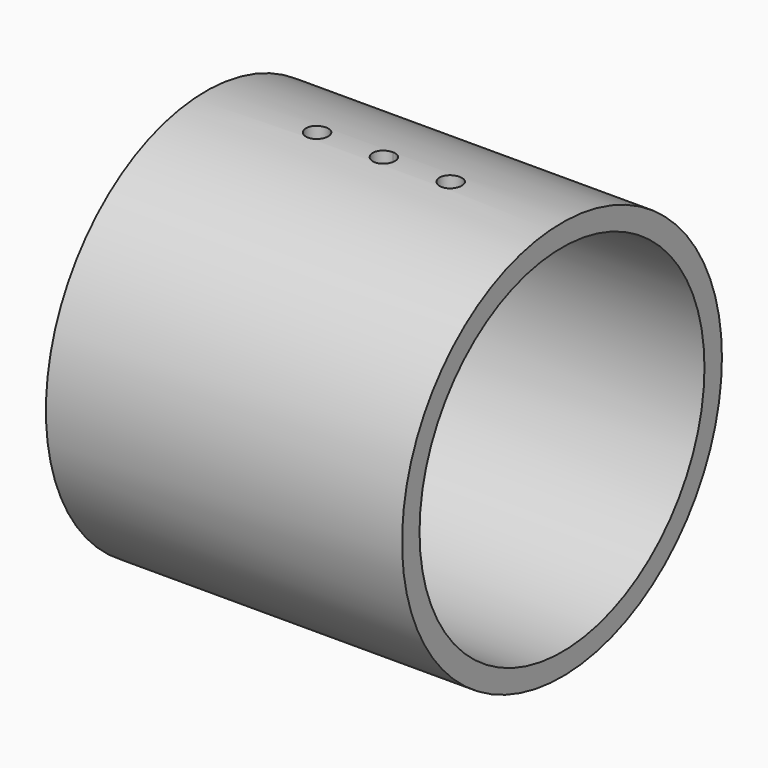
from build123d import *

# Parameters (mm, degrees)
F0_R     = 57.023
F0_R_2   = 50.8
F1_DEPTH = 101.6
F3_DEPTH = 127


# Not quite as in the source:
# - a pattern or mirror of a feature is missing from the dataset's text; its kind, count and spacing are read off the source's solid


with BuildPart() as f1:
    # F0 (on Right) → F1 (new body)
    with BuildSketch(Plane.YZ):
        Circle(F0_R)
        Circle(F0_R_2, mode=Mode.SUBTRACT)
    extrude(amount=F1_DEPTH)

    # F2 (on Top) → F3 (cut)
    with BuildSketch(Plane.XY):
        with BuildLine():
            ThreePointArc((53.975, 0), (50.8, 3.175), (47.625, 0))
            Line((47.625, 0), (53.975, 0))
        make_face()
        with BuildLine():
            Line((53.975, 0), (47.625, 0))
            ThreePointArc((47.625, 0), (50.8, -3.175), (53.975, 0))
        make_face()
        with BuildLine():
            ThreePointArc((73.025, 0), (69.85, 3.175), (66.675, 0))
            Line((66.675, 0), (73.025, 0))
        make_face()
        with BuildLine():
            Line((73.025, 0), (66.675, 0))
            ThreePointArc((66.675, 0), (69.85, -3.175), (73.025, 0))
        make_face()
    f3 = extrude(amount=F3_DEPTH, mode=Mode.SUBTRACT)

    # F3_copies: F3 across plane
    add(f3.mirror(Plane(origin=(50.800012, -2e-06, 1.1e-05), x_dir=(0, 0, -1), z_dir=(-1, 0, 0))), mode=Mode.SUBTRACT)


solid = f1.part
